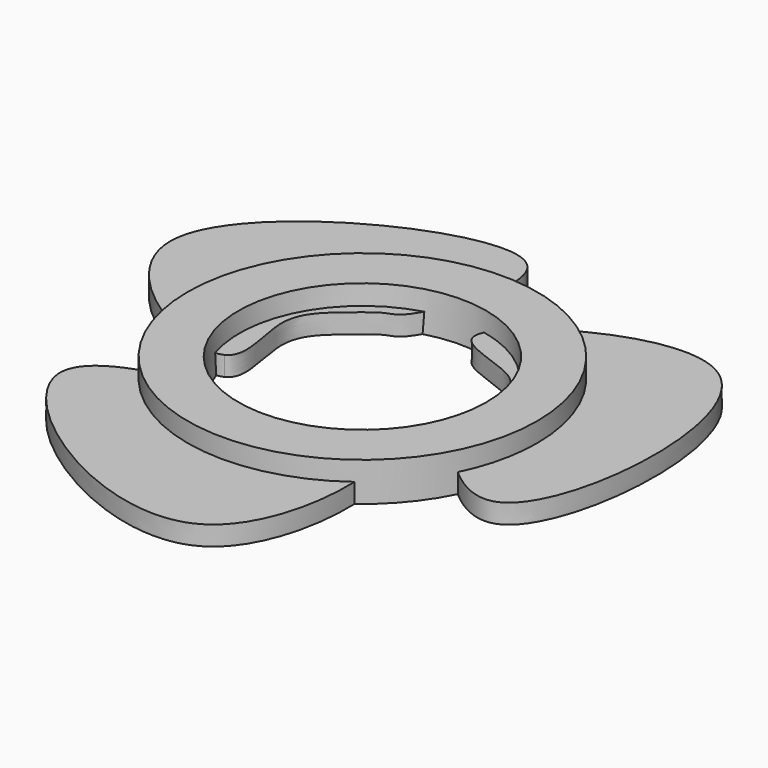
from build123d import *

# Parameters (mm, degrees)
F0_R            = 31.4965218055
F0_R_2          = 21.9661022679
F1_DEPTH        = 7
F2_DEPTH        = 7
F3_DEPTH        = 25
F3_TAPER        = -3
F5_DEPTH        = 3.5
F5_COPIES_COUNT = 3


# Not quite as in the source:
# - a pattern or mirror of a feature is missing from the dataset's text; its kind, count and spacing are read off the source's solid


with BuildPart() as f1:
    # F0 (on Top) → F1 (new body)
    with BuildSketch(Plane.XY):
        Circle(F0_R)
        Circle(F0_R_2, mode=Mode.SUBTRACT)
    extrude(amount=F1_DEPTH)

    # F0 (on Top) → F2 (join)
    with BuildSketch(Plane.XY):
        Circle(F0_R_2)
    extrude(amount=F2_DEPTH)

    # F0 (on Top) → F3 (cut)
    with BuildSketch(Plane.XY):
        Circle(F0_R_2)
    extrude(amount=F3_DEPTH, taper=F3_TAPER, mode=Mode.SUBTRACT)

    # F4 (on Top) → F5 (join)
    with BuildSketch(Plane.XY):
        with BuildLine():
            add(Edge.make_bspline(
                [(4.2096277725, 20.3023137728), (4.6555030942, 26.2130886173), (53.0558186012, 55.9434326796), (46.2627887272, -38.1346327884), (18.6182602641, -3.5763383948), (20.6867763474, -0.2501628504), (19.4263878886, 5.813657059), (17.971378958, 15.3421738211), (3.9401302616, 16.7297027086), (4.2096277725, 20.3023137728)],
                knots=[0, 0, 0, 0, 0.2082520051, 0.4547442195, 0.6201159064, 0.6875373762, 0.769587335, 0.8741275997, 1, 1, 1, 1], degree=3))
        make_face()
    f5 = extrude(amount=F5_DEPTH)

    # F5_copies: F5 ×3 about axis
    f5_copies_axis = Axis((0, 0, 0), (0, 0, 1))
    for i in range(1, F5_COPIES_COUNT):
        add(f5.rotate(f5_copies_axis, i * 360 / F5_COPIES_COUNT))


solid = f1.part
